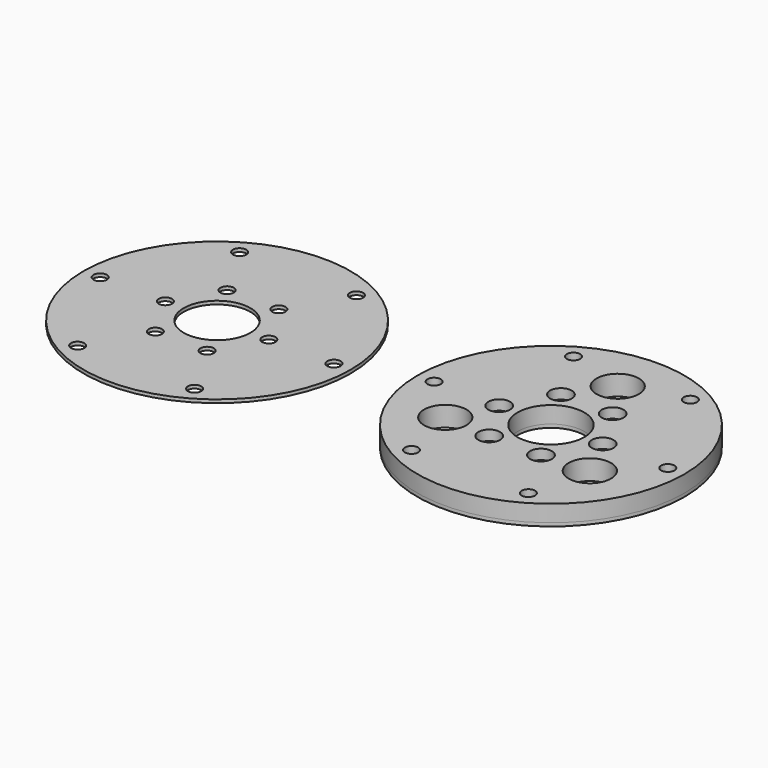
from build123d import *

# Parameters (mm, degrees)
F0_R           = 40
F0_R_2         = 30
F1_DEPTH       = 1
F2_D           = 4
F3_D           = 20
F5_DEPTH       = 5
F7_D           = 3.15
F7_CBORE_D     = 6.5
F7_CBORE_DEPTH = 3
F9_D           = 12.7


# Not quite as in the source:
# - a feature names something its author has since deleted; it is built from what else it names


with BuildPart() as f1:
    # F0 (on Top) → F1 (new body)
    with BuildSketch(Plane.XY):
        Circle(F0_R)
        Circle(F0_R_2, mode=Mode.SUBTRACT)
        Circle(F0_R_2)
    extrude(amount=-F1_DEPTH)

    # F2 (through all)
    with Locations(Plane.XY):
        with Locations((35, 0), (17.5, 30.3108891325), (-17.5, 30.3108891325), (-35, 0), (-17.5, -30.3108891325), (17.5, -30.3108891325), (-7.75, -13.4233937587), (7.75, -13.4233937587), (15.5, 0), (7.75, 13.4233937587), (-7.75, 13.4233937587), (-15.5, 0)):
            Hole(F2_D / 2)

    # F3 (through all)
    with Locations(Plane.XY):
        with Locations((0, 0)):
            Hole(F3_D / 2)


with BuildPart() as f4_1:
    # F4: copy of F1
    add(f1.part.moved(Location((100, 0, 0))))

    # F5 (add): a face of the model
    f5_faces = [f4_1.faces().sort_by_distance(p)[0] for p in [
        (61.1313708499, 0, 0),
    ]]
    extrude(f5_faces, amount=F5_DEPTH)

    # F7 (through all)
    with Locations(Plane.XY.offset(5)):
        with Locations((115.5, 0), (107.75, -13.4233937587), (92.25, -13.4233937587), (84.5, 0), (92.25, 13.4233937587), (107.75, 13.4233937587)):
            CounterBoreHole(F7_D / 2, F7_CBORE_D / 2, F7_CBORE_DEPTH)

    # F9 (through all)
    with Locations(Plane.XY.offset(5)):
        with Locations((100, 25), (121.6506350946, -12.5), (78.3493649054, -12.5)):
            Hole(F9_D / 2)


solid = Compound([f1.part, f4_1.part])
